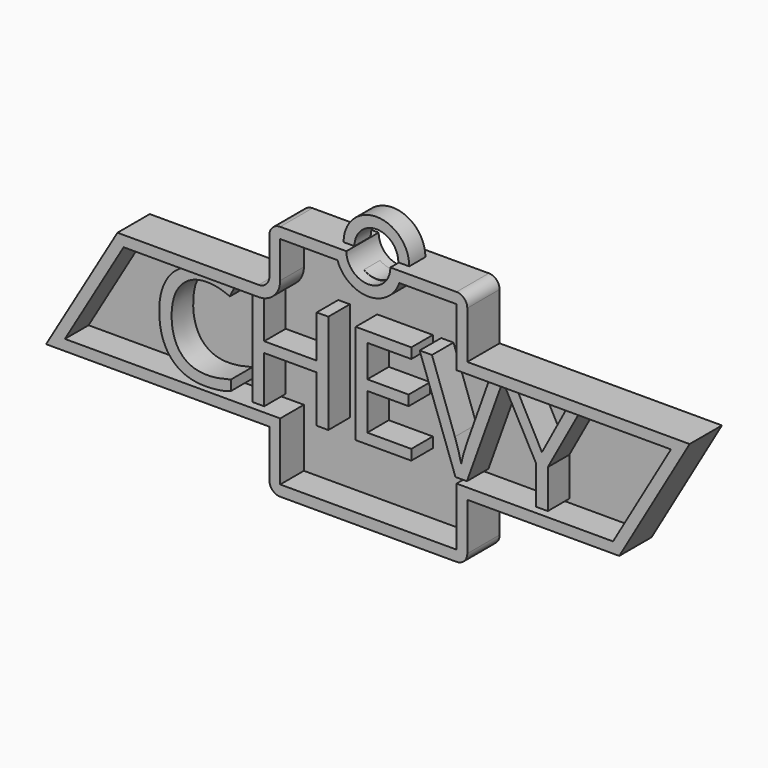
from build123d import *

# Parameters (mm, degrees)
F1_DEPTH     = 9.525
F2_R         = 2.54
F3_T         = 2.54
F3_T3_DEPTH  = 14.605
F6_R         = 7.7450232811
F7_DEPTH     = 2.38125
F8_TEXT_SIZE = 32.9695357424
F9_DEPTH     = 6.35


# Not quite as in the source:
# - a shell that OpenCascade refuses in one call is made with other operations: the cavity is built on its own and cut out
# - Text() gives the source's letters only with a copy of the font that has no kerning and outlines rounded to 1/6400 em; it was checked with that copy


with BuildPart() as f1:
    # F0 (on Front) → F1 (new body)
    with BuildSketch(Plane.XZ):
        with BuildLine():
            Line((75.7989436388, 14.3175795674), (59.195369482, 14.3175795674))
            Line((59.195369482, 14.3175795674), (23.3412608504, 14.3175795674))
            Line((23.3412608504, 14.3175795674), (23.3412608504, 28.033580631))
            Line((23.3412608504, 28.033580631), (6.2564210966, 28.033580631))
            Line((6.2564210966, 28.033580631), (5.4156100894, 28.033580631))
            Line((5.4156100894, 28.033580631), (5.1908632253, 28.033580631))
            ThreePointArc((5.1908632253, 28.033580631), (0, 22.8427174057), (-5.1908632253, 28.033580631))
            Line((-5.1908632253, 28.033580631), (-6.4970520325, 28.033580631))
            Line((-6.4970520325, 28.033580631), (-23.3412608504, 28.033580631))
            Line((-23.3412608504, 28.033580631), (-23.3412608504, 14.3175795674))
            Line((-23.3412608504, 14.3175795674), (-59.195369482, 14.3175795674))
            Line((-59.195369482, 14.3175795674), (-76.0395824909, -14.3175795674))
            Line((-76.0395824909, -14.3175795674), (-59.195369482, -14.3175795674))
            Line((-59.195369482, -14.3175795674), (-23.3412608504, -14.3175795674))
            Line((-23.3412608504, -14.3175795674), (-23.3412608504, -28.033580631))
            Line((-23.3412608504, -28.033580631), (23.3412608504, -28.033580631))
            Line((23.3412608504, -28.033580631), (23.3412608504, -14.3175795674))
            Line((23.3412608504, -14.3175795674), (59.195369482, -14.3175795674))
            Line((59.195369482, -14.3175795674), (75.7989436388, 14.3175795674))
        make_face()
    extrude(amount=F1_DEPTH)

    # F2
    f2_edges = [f1.edges().sort_by_distance(p)[0] for p in [
        (23.341261, -4.7625, 28.033581),
        (23.341261, -4.7625, -28.033581),
        (-23.341261, -4.7625, -28.033581),
        (-23.341261, -4.7625, 14.31758),
        (-23.341261, -4.7625, 28.033581),
    ]]
    fillet(f2_edges, radius=F2_R)

    # F3: shell of thickness 2.54, made by hand


with BuildPart() as f3_core1:
    # F3_t2: copy of F1
    add(f1.part)

    # the walls: a layer under each face that stays
    f3_faces = [f3_core1.faces().sort_by_distance(p)[0] for p in [
        (-0.1203194261, 0, 0),
        (-23.3412608504, -4.7625, -19.9055800992),
        (-49.6904216707, -4.7625, -14.3175795674),
        (0, -4.7625, -28.033580631),
        (-67.6174759865, -4.7625, 0),
        (-42.5383151662, -4.7625, 14.3175795674),
        (23.3412608504, -4.7625, -19.9055800992),
        (-24.0852096262, -4.7625, 15.0615283432),
        (41.2683151662, -4.7625, -14.3175795674),
        (-23.3412608504, -4.7625, 21.1755800992),
        (67.4971565604, -4.7625, 0),
        (49.5701022446, -4.7625, 14.3175795674),
        (-12.9960620379, -4.7625, 28.033580631),
        (23.3412608504, -4.7625, 19.9055800992),
        (0, -4.7625, 22.8427174057),
        (12.9960620379, -4.7625, 28.033580631),
    ]]
    thicken(f3_faces, amount=-F3_T, mode=Mode.SUBTRACT)

    # F3_s4 → F3_t3 (cut)
    with BuildSketch(Plane.XZ.offset(-2.54)):
        Polygon((-23.3666608504, -14.3429795674), (-20.8012608504, -14.3175795674), (-20.8012608504, -11.7775795674), (-23.3412608504, -11.7775795674), align=None)
        Polygon((23.3666608504, -14.3429795674), (20.8012608504, -14.3175795674), (20.8012608504, -11.7775795674), (23.3412608504, -11.7775795674), align=None)
        Polygon((23.3666608504, 14.3429795674), (23.3412608504, 11.7775795674), (20.8012608504, 11.7775795674), (20.8012608504, 14.3175795674), align=None)
    extrude(amount=F3_T3_DEPTH, mode=Mode.SUBTRACT)


with BuildPart() as f1_1:
    add(f1.part)

    # what is left inside the walls is the cavity
    f3_cavity = [f3_core1.part.solids().sort_by_distance(p)[0] for p in [
        (-0.104264, -2.5654, -8.49786),
    ]]
    add(f3_cavity, mode=Mode.SUBTRACT)

    # F6 (on offset) → F7 (join, symmetric)
    with BuildSketch(Plane.XZ.offset(4.6355)):
        with Locations((-0.1059737988, 28.082979843)):
            Circle(F6_R)
        with BuildLine():
            ThreePointArc((-5.2751202321, 28.082979843), (-0.1059737988, 33.2521262764), (5.0631726346, 28.082979843))
            ThreePointArc((5.0631726346, 28.082979843), (-0.1059737988, 22.9138334097), (-5.2751202321, 28.082979843))
        make_face(mode=Mode.SUBTRACT)
    extrude(amount=F7_DEPTH, both=True)

    # F8 (on face) → F9 (join)
    with BuildSketch(Plane.XZ.offset(2.54)):
        with Locations((-51.8624521792, -10.9132146463)):
            Text('CHEVY', F8_TEXT_SIZE, font='Open Sans', text_align=(TextAlign.LEFT, TextAlign.BOTTOM))
    extrude(amount=F9_DEPTH)


solid = f1_1.part
